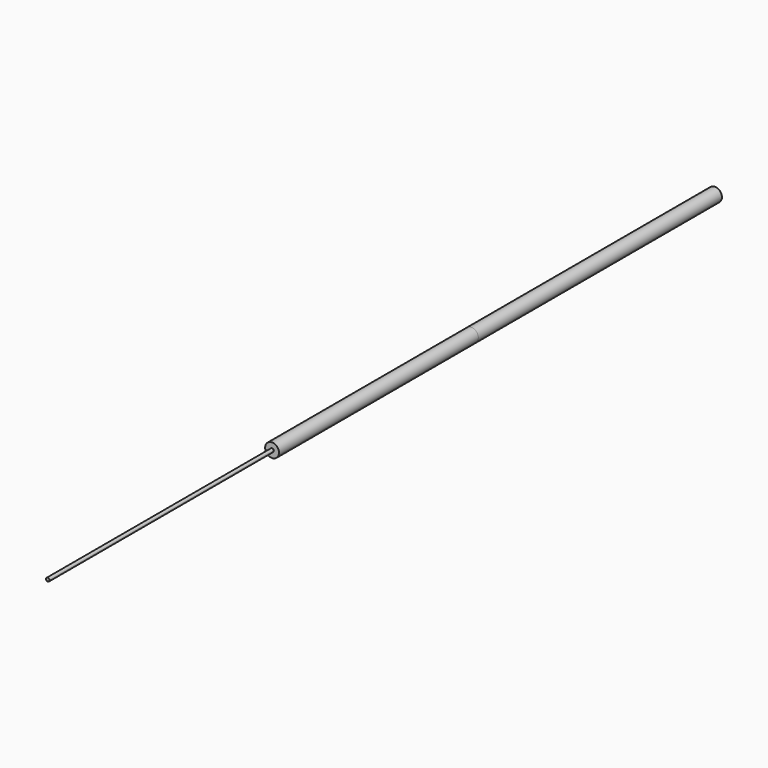
from build123d import *

# Parameters (mm, degrees)
F0_R       = 25.4
F1_DEPTH   = 914.4
F1_FACE1_R = 25.4
F2_R       = 6.35
F3_DEPTH   = 1028.69492
F4_R       = 6.35
F5_DEPTH   = 1028.69492
F6_R       = 25.4
F6_R_2     = 6.35
F7_DEPTH   = 1117.6


# Not quite as in the source:
# - an extrude ends at something that could not be found from the text; its depth is read off the source's solid


with BuildPart() as f1:
    # F0 (on Front) → F1 (new body)
    with BuildSketch(Plane.XZ):
        with Locations((-45.4621687531, 36.2614989281)):
            Circle(F0_R)
    extrude(amount=F1_DEPTH)

    # F1_face1 (on face) + F2 (on face) → F3 (cut, through all)
    with BuildSketch(Plane(origin=(-45.4621687531, -914.4, 36.2614989281), x_dir=(1, 0, 0), z_dir=(0, -1, 0))):
        Circle(F1_FACE1_R)
    with BuildSketch(Plane(origin=(0, 0, 0), x_dir=(-1, 0, 0), z_dir=(0, 1, 0))):
        with Locations((45.4621687531, 36.2614989281)):
            Circle(F2_R)
    extrude(amount=F3_DEPTH, dir=(0, -1, 0), mode=Mode.SUBTRACT)


with BuildPart() as f5:
    # F4 (on face) → F5 (new body)
    with BuildSketch(Plane.XZ.offset(914.4)):
        with Locations((-45.4621687531, 36.2614989281)):
            Circle(F4_R)
    extrude(amount=F5_DEPTH)


with BuildPart() as f7:
    # F6 (on face) → F7 (new body)
    with BuildSketch(Plane(origin=(0, 0, 0), x_dir=(-1, 0, 0), z_dir=(0, 1, 0))):
        with Locations((45.4621687531, 36.2614989281)):
            Circle(F6_R)
        with Locations((45.4621687531, 36.2614989281)):
            Circle(F6_R_2, mode=Mode.SUBTRACT)
    extrude(amount=F7_DEPTH)


solid = Compound([f1.part, f5.part, f7.part])
